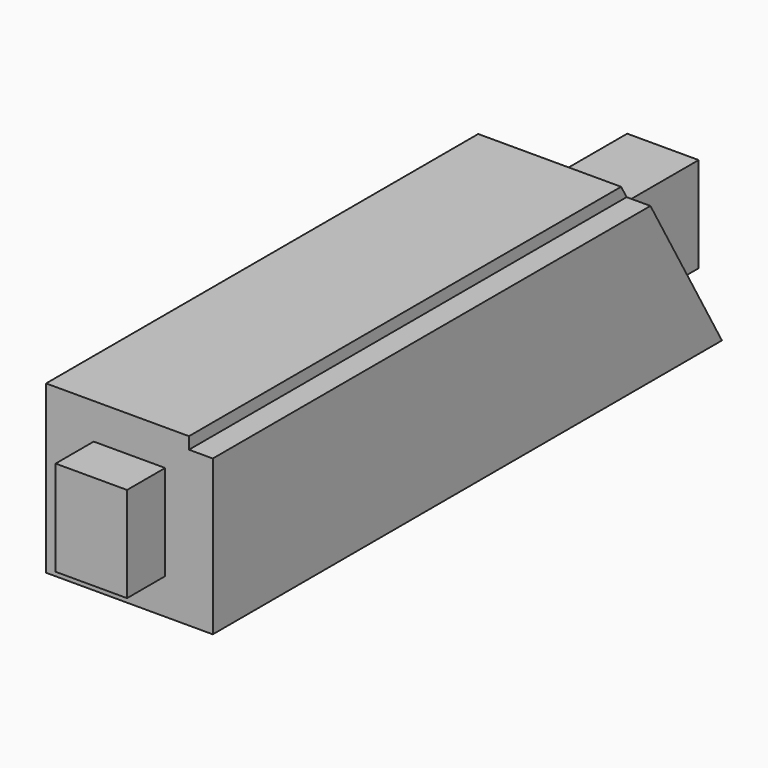
from build123d import *

# Parameters (mm, degrees)
F0_W     = 381
F0_H     = 88.9
F1_DEPTH = 44.45
F4_W     = 12.7
F4_H     = 6.35
F5_DEPTH = 381.001
F6_W     = 88.9
F6_H     = 88.9
F6_W_2   = 38.1
F6_H_2   = 50.8
F7_REACH = 193.287585695
F8_W     = 88.9
F8_H     = 88.9
F8_W_2   = 38.1
F8_H_2   = 50.8
F9_DEPTH = 25.4


with BuildPart() as f1:
    # F0 (on Right) → F1 (new body, symmetric)
    with BuildSketch(Plane.YZ):
        Rectangle(F0_W, F0_H)
    extrude(amount=F1_DEPTH, both=True)

    # F4 (on face) → F5 (cut, through all)
    with BuildSketch(Plane(origin=(0, 190.5, 0), x_dir=(-1, 0, 0), z_dir=(0, 1, 0))):
        with Locations((-38.1, 41.275)):
            Rectangle(F4_W, F4_H)
    extrude(amount=-F5_DEPTH, mode=Mode.SUBTRACT)

    f7_end = Plane(origin=(0, 111.4494145991, 64.3453495198), x_dir=(0, -0.5, 0.8660254038), z_dir=(0, 0.8660254038, 0.5))
    # F6 (on face) → F7 (cut, up to a plane its end follows)
    with BuildSketch(Plane(origin=(0, 190.5, 0), x_dir=(-1, 0, 0), z_dir=(0, 1, 0))):
        Rectangle(F6_W, F6_H)
        Rectangle(F6_W_2, F6_H_2, mode=Mode.SUBTRACT)
    f7_long = extrude(amount=-F7_REACH, mode=Mode.PRIVATE)
    add(split(f7_long, bisect_by=f7_end, keep=Keep.TOP, mode=Mode.PRIVATE), mode=Mode.SUBTRACT)

    # F8 (on face) → F9 (cut)
    with BuildSketch(Plane.XZ.offset(190.5)):
        Rectangle(F8_W, F8_H)
        Rectangle(F8_W_2, F8_H_2, mode=Mode.SUBTRACT)
    extrude(amount=-F9_DEPTH, mode=Mode.SUBTRACT)


solid = f1.part
